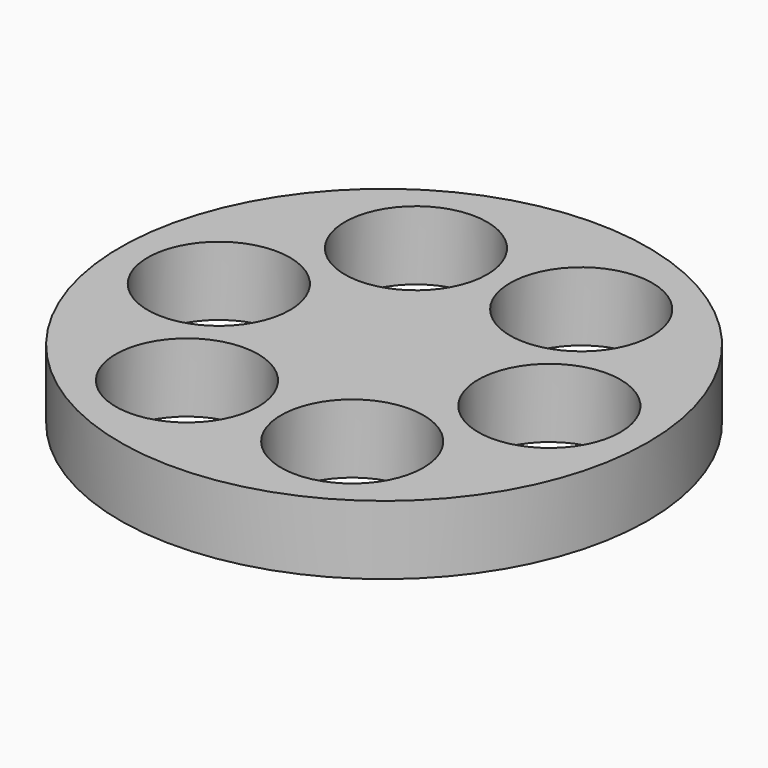
from build123d import *

# Parameters (mm, degrees)
F0_R     = 57.5
F0_R_2   = 15.5
F1_DEPTH = 15


# Not quite as in the source:
# - a feature of the source that left no trace in its solid (it failed there, or was rolled back) is left out


with BuildPart() as f1:
    # F0 (on Top) → F1 (new body)
    with BuildSketch(Plane.XY):
        Circle(F0_R)
        with Locations((-18.0000001252, -31.1769144639)):
            Circle(F0_R_2, mode=Mode.SUBTRACT)
        with Locations((17.9999998998, -31.1769145941)):
            Circle(F0_R_2, mode=Mode.SUBTRACT)
        with Locations((36, -8.68e-08)):
            Circle(F0_R_2, mode=Mode.SUBTRACT)
        with Locations((-36, 0)):
            Circle(F0_R_2, mode=Mode.SUBTRACT)
        with Locations((-17.999999975, 31.1769145507)):
            Circle(F0_R_2, mode=Mode.SUBTRACT)
        with Locations((18.0000000501, 31.1769145073)):
            Circle(F0_R_2, mode=Mode.SUBTRACT)
    extrude(amount=F1_DEPTH)


solid = f1.part
